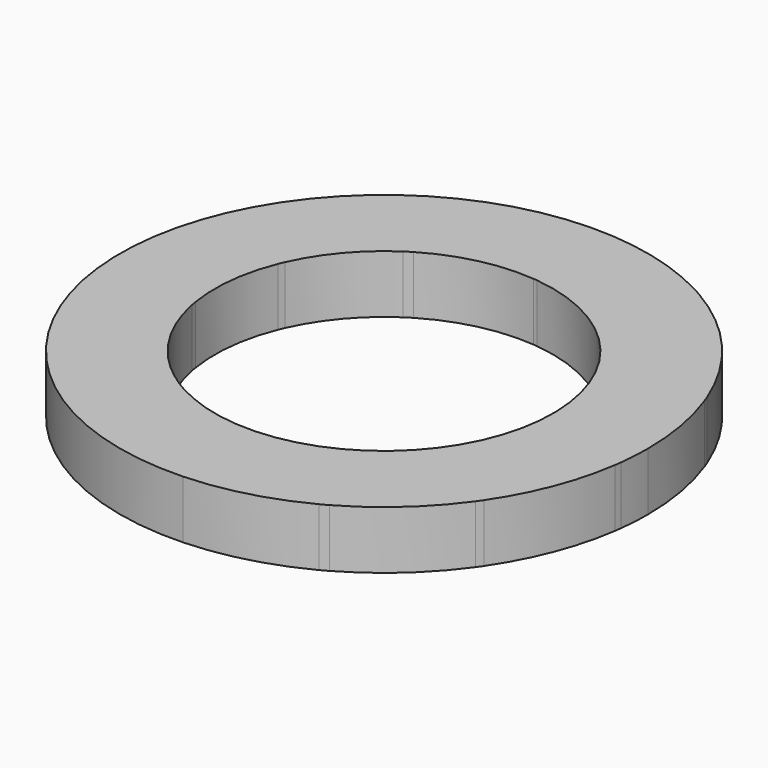
from build123d import *

# Parameters (mm, degrees)
F1_DEPTH = 5.1


with BuildPart() as f1:
    # F0 (on Top) → F1 (new body)
    with BuildSketch(Plane.XY):
        with BuildLine():
            ThreePointArc((23.0623797864, -2.752888696), (23.1851344055, -1.378876421), (23.2261007831, 0))
            ThreePointArc((23.2261007831, 0), (22.8721340644, 4.039460475), (21.8210228424, 7.9557978667))
            ThreePointArc((21.8210228424, 7.9557978667), (21.7129320627, 8.2462317956), (21.600975855, 8.5351976954))
            ThreePointArc((21.600975855, 8.5351976954), (17.6168585154, 15.135985387), (11.6914938176, 20.0688995687))
            ThreePointArc((11.6914938176, 20.0688995687), (11.3296656288, 20.2753652082), (10.9641925592, 20.4753080346))
            ThreePointArc((10.9641925592, 20.4753080346), (6.4344525637, 22.3170243938), (1.6195142321, 23.1695690775))
            ThreePointArc((1.6195142321, 23.1695690775), (-23.2232414227, 0.3644384862), (0.891703377, -23.2089772001))
            ThreePointArc((0.891703377, -23.2089772001), (5.9586225424, -22.4487544194), (10.7355743028, -20.5960967655))
            ThreePointArc((10.7355743028, -20.5960967655), (11.0730407687, -20.4166482489), (11.4075086171, -20.231670834))
            ThreePointArc((11.4075086171, -20.231670834), (15.509940512, -17.2885367484), (18.8794446221, -13.5284266767))
            ThreePointArc((18.8794446221, -13.5284266767), (19.0526450726, -13.283390882), (19.2226654093, -13.0361379307))
            ThreePointArc((19.2226654093, -13.0361379307), (21.6572092153, -8.3914865543), (22.9877271358, -3.3190599146))
            ThreePointArc((22.9877271358, -3.3190599146), (23.0267936185, -3.0362037542), (23.0623797864, -2.752888696))
        make_face()
        with BuildLine():
            ThreePointArc((-7.6265143045, 12.7618767873), (-3.3183069466, 14.491999813), (1.3134897969, 14.8089150219))
            ThreePointArc((1.3134897969, 14.8089150219), (1.4665804544, 14.7945382268), (1.6195142321, 14.7785788635))
            ThreePointArc((1.6195142321, 14.7785788635), (11.0703798721, 9.9235028624), (14.8670514754, 0))
            ThreePointArc((14.8670514754, 0), (7.4772282889, -12.8499134895), (-7.3458637029, -12.9254596062))
            ThreePointArc((-7.3458637029, -12.9254596062), (-7.689867558, -12.7238027536), (-8.0283394714, -12.5129926438))
            ThreePointArc((-8.0283394714, -12.5129926438), (-9.5257186584, -11.4144602856), (-10.874459487, -10.1378178341))
            ThreePointArc((-10.874459487, -10.1378178341), (-11.0561755007, -9.9393260772), (-11.2342689854, -9.7375777243))
            ThreePointArc((-11.2342689854, -9.7375777243), (-13.3519365266, -6.5387315713), (-14.5805712978, -2.9045068776))
            ThreePointArc((-14.5805712978, -2.9045068776), (-14.6272984034, -2.6592030743), (-14.6698988149, -2.4131490494))
            ThreePointArc((-14.6698988149, -2.4131490494), (-14.7754620576, 1.6477076674), (-13.7779120757, 5.5855490693))
            ThreePointArc((-13.7779120757, 5.5855490693), (-13.6764347777, 5.8296098793), (-13.570634607, 6.0718280554))
            ThreePointArc((-13.570634607, 6.0718280554), (-11.3456382043, 9.6075862374), (-8.2248041845, 12.3847412448))
            ThreePointArc((-8.2248041845, 12.3847412448), (-7.9279021351, 12.57686715), (-7.6265143045, 12.7618767873))
        make_face(mode=Mode.SUBTRACT)
    extrude(amount=F1_DEPTH)


solid = f1.part
